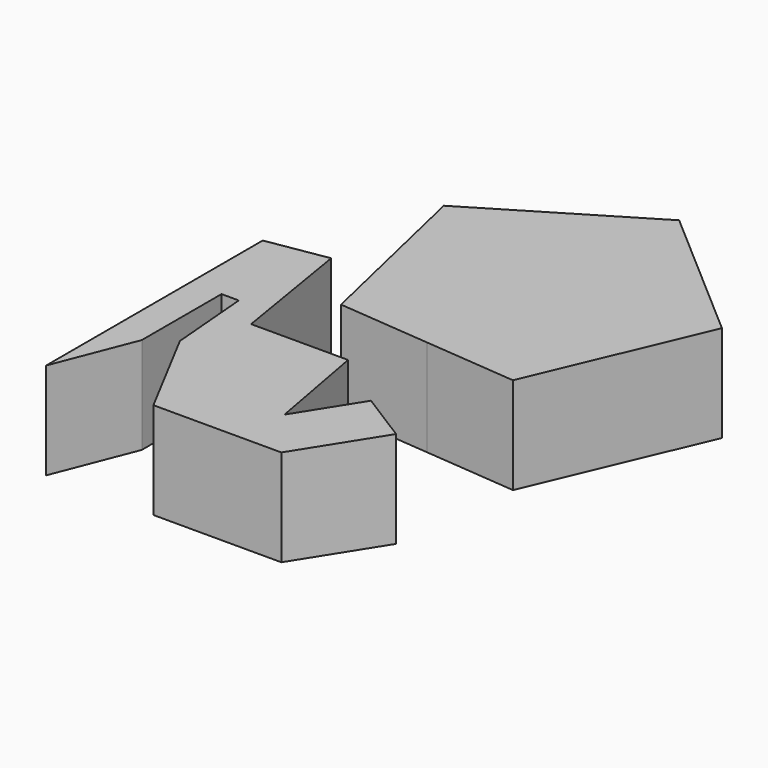
from build123d import *

# Parameters (mm, degrees)
F1_DEPTH = 25.4
F5_DEPTH = 25.4


# Not quite as in the source:
# - the program builds the solid bodies; features that only make, move or delete a surface that nothing else refers to are left out


with BuildPart() as f1:
    # F0 (on Top) → F1 (new body)
    with BuildSketch(Plane.XY):
        Polygon((-9.2521887273, 24.9605737627), (12.1087450534, -10.5494055897), (21.6147225683, 11.8767181747), align=None)
        Polygon((-12.1572746882, -8.4387370915), (12.1087450534, -10.5494055897), (-9.2521887273, 24.9605737627), align=None)
        Polygon((-36.4232944299, -6.3280685934), (-12.1572746882, -8.4387370915), (-9.2521887273, 24.9605737627), align=None)
        Polygon((-9.2521887273, 24.9605737627), (21.6147225683, 11.8767181747), (31.1207000832, 34.3028419391), align=None)
        Polygon((-41.914541887, 17.4025200419), (-9.2521887273, 24.9605737627), (-47.4057893441, 41.1331086771), align=None)
        Polygon((-26.5335471715, 53.6887505286), (-9.2521887273, 24.9605737627), (-5.661304999, 66.2443923801), align=None)
        Polygon((-5.661304999, 66.2443923801), (-9.2521887273, 24.9605737627), (12.7296975421, 50.2736171596), align=None)
        Polygon((12.7296975421, 50.2736171596), (-9.2521887273, 24.9605737627), (31.1207000832, 34.3028419391), align=None)
        Polygon((-36.4232944299, -6.3280685934), (-9.2521887273, 24.9605737627), (-41.914541887, 17.4025200419), align=None)
        Polygon((-47.4057893441, 41.1331086771), (-9.2521887273, 24.9605737627), (-26.5335471715, 53.6887505286), align=None)
    extrude(amount=F1_DEPTH)


with BuildPart() as f5:
    # F4 (on Top) → F5 (new body)
    with BuildSketch(Plane.XY):
        Polygon((-53.9466738701, -17.9940983653), (-52.1350763738, -39.5913757384), (-38.5621264577, -65.2649849653), (-4.9518779851, -65.2649849653), (8.3174398169, -44.1713742912), (-4.9518779851, -35.8240696191), (-14.9513309923, -51.7197299563), (-19.9307296425, -24.6265847236), (-45.4155802727, -24.6265847236), (-50.8631318808, 8.4827328101), (-66.7493829843, 5.868931645), (-66.7493829843, -65.2649849653), (-58.4871545434, -44.1713742912), (-58.4871545434, -17.9940983653), align=None)
    extrude(amount=F5_DEPTH)


solid = Compound([f1.part, f5.part])
